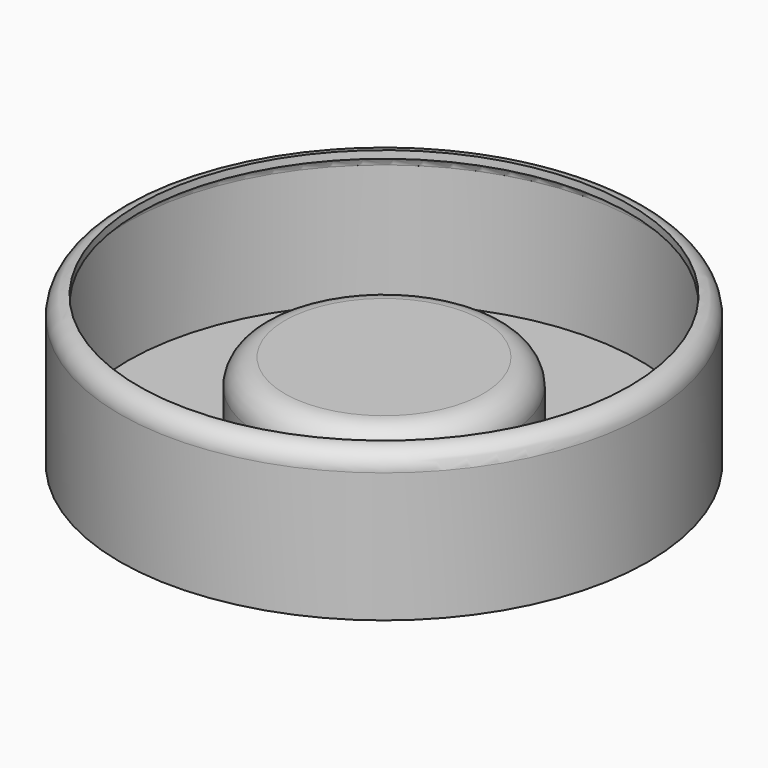
from build123d import *

# Parameters (mm, degrees)
F2_T = 2.54
F3_R = 5.08


# Not quite as in the source:
# - a shell that OpenCascade refuses in one call is made with other operations: the cavity is built on its own and cut out


with BuildPart() as f1:
    # F0 (on Front) → F1 (revolve)
    with BuildSketch(Plane.XZ):
        with BuildLine():
            ThreePointArc((-57.9764892951, 60.004751325), (-62.3916472883, 58.1048437598), (-64.2108023167, 53.6558052296))
            Line((-64.2108023167, 53.6558052296), (-64.2108023167, 9.8601095378))
            Line((-64.2108023167, 9.8601095378), (-14.9272382259, 9.8601095378))
            Line((-14.9272382259, 9.8601095378), (-14.9272382259, 32.7742578626))
            ThreePointArc((-14.9272382259, 32.7742578626), (-13.0673662865, 37.2643859231), (-8.5772382259, 39.1242578626))
            Line((-8.5772382259, 39.1242578626), (24.8787216842, 39.1242578626))
            Line((24.8787216842, 39.1242578626), (24.8787216842, 61.514493078))
            Line((24.8787216842, 61.514493078), (-57.9764892951, 60.004751325))
        make_face()
    revolve(axis=Axis((24.8787216842, 0, 50.3193754703), (0, 0, 1)))

    # F2: shell of thickness 2.54, made by hand


with BuildPart() as f2_core1:
    # F2_t2: copy of F1
    add(f1.part)

    # the walls: a layer under each face that stays
    f2_faces = [f2_core1.faces().sort_by_distance(p)[0] for p in [
        (112.1490906567, 0, 58.1048437598),
        (113.9682456851, 0, 31.7579573837),
        (84.2717376848, 59.3930160006, 9.8601095378),
        (64.6846815944, 0, 21.3171837002),
        (62.8248096549, 0, 37.2643859231),
        (24.8787216842, 0, 39.1242578626),
    ]]
    thicken(f2_faces, amount=-F2_T, mode=Mode.SUBTRACT)


with BuildPart() as f1_1:
    add(f1.part)

    # what is left inside the walls is the cavity
    f2_cavity = [f2_core1.part.solids().sort_by_distance(p)[0] for p in [
        (111.402846, 0, 39.903907),
    ]]
    add(f2_cavity, mode=Mode.SUBTRACT)

    # F3
    f3_edges = [f1_1.edges().sort_by_distance(p)[0] for p in [
        (64.684682, 0, 9.86011),
    ]]
    fillet(f3_edges, radius=F3_R)


solid = f1_1.part
